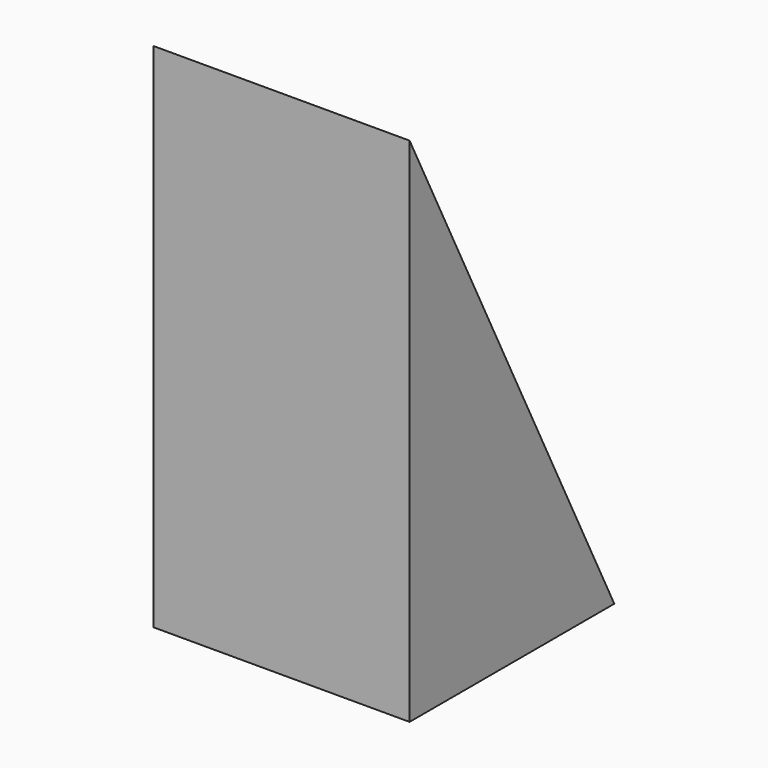
from build123d import *

# Parameters (mm, degrees)
F0_W     = 15
F0_H     = 15
F1_DEPTH = 30
F3_DEPTH = 25
F4_R     = 4
F5_DEPTH = 10


# Not quite as in the source:
# - a feature names something its author has since deleted; it is built from what else it names


with BuildPart() as f1:
    # F0 (on Top) → F1 (new body)
    with BuildSketch(Plane.XY):
        with Locations((7.5, 7.5)):
            Rectangle(F0_W, F0_H)
    extrude(amount=F1_DEPTH)

    # F2 (on face) → F3 (cut)
    with BuildSketch(Plane.YZ.offset(15)):
        Polygon((15, 30), (0, 30), (15, 0), align=None)
    extrude(amount=-F3_DEPTH, mode=Mode.SUBTRACT)

    # F4 (on face) → F5 (cut)
    with BuildSketch(Plane(origin=(0, 0, 0), x_dir=(1, 0, 0), z_dir=(0, 0, -1))):
        with Locations((7.5, -5.5)):
            Circle(F4_R)
    extrude(amount=-F5_DEPTH, mode=Mode.SUBTRACT)


solid = f1.part
